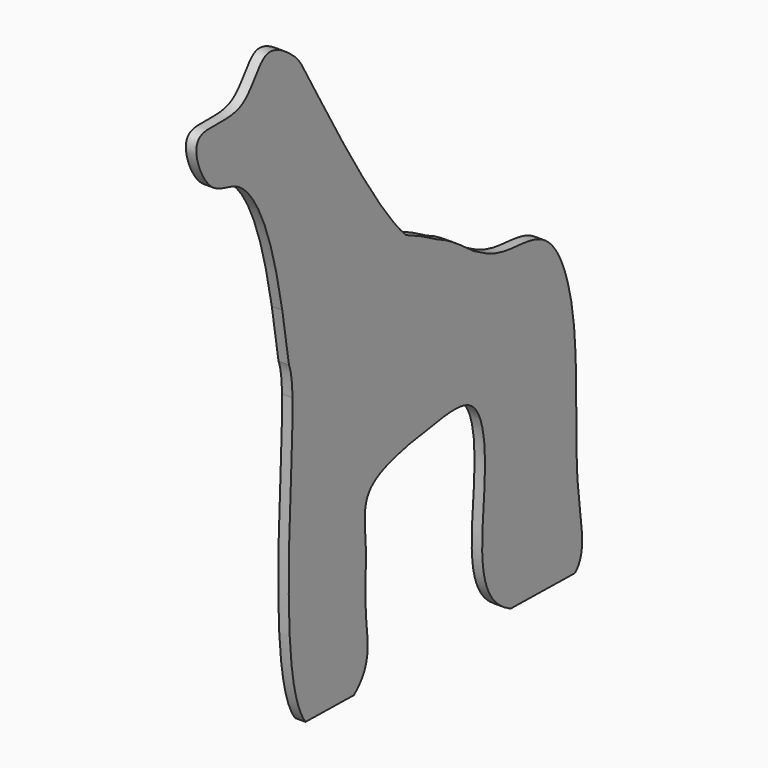
from build123d import *

# Parameters (mm, degrees)
F1_DEPTH = 12


with BuildPart() as f1:
    # F0 (on Right) → F1 (new body)
    with BuildSketch(Plane.YZ):
        with BuildLine():
            add(Edge.make_bspline(
                [(-178.4369833225, -144.2066091912), (-219.218467925, -89.3323742164), (-195.3415795005, 113.7315380775), (-197.007060051, 190.3274804354)],
                knots=[0.0031505946, 0.0031505946, 0.0031505946, 0.0031505946, 0.0998386573, 0.0998386573, 0.0998386573, 0.0998386573], degree=3))
            Line((-178.4369833225, -144.2066091912), (-109.1511381578, -145.4286668255))
            add(Edge.make_bspline(
                [(115.2884357666, -149.3873122617), (107.1403709504, -145.3507189429), (62.2417659614, -114.3804366066), (86.2834183467, -3.0492512147), (70.8695963558, 91.374454728), (0.4418432139, 80.4667572796), (-101.9293868506, 65.0970756202), (-88.6503884924, -2.5844560488), (-96.59431316, -67.481945255), (-83.1150537691, -119.8184104695), (-104.8879154969, -142.055068639), (-109.1511381578, -145.4286668255)],
                knots=[0.6073825493, 0.6073825493, 0.6073825493, 0.6073825493, 0.6195734428, 0.6825204089, 0.7308072739, 0.7727612584, 0.824213165, 0.8635812279, 0.9083971983, 0.9523997564, 0.9613925241, 0.9613925241, 0.9613925241, 0.9613925241], degree=3))
            Line((115.2884357666, -149.3873122617), (207.5685221579, -151.0149402974))
            add(Edge.make_bspline(
                [(63.0940198898, 232.5838804245), (82.5887469223, 220.8525880353), (109.669328549, 211.0698213252), (178.2811116459, 213.9353754027), (217.1880000792, 96.1874140131), (202.5402479992, -58.3272921235), (224.9464188994, -135.8202031967), (207.5685221579, -151.0149402974)],
                knots=[0.3062619929, 0.3062619929, 0.3062619929, 0.3062619929, 0.3456878235, 0.3855453305, 0.441597856, 0.5123533056, 0.5605055591, 0.5605055591, 0.5605055591, 0.5605055591], degree=3))
            add(Edge.make_bspline(
                [(10.2934252514, 265.8684253693), (30.8960203842, 253.7377434197), (48.6497019648, 241.2760009482), (63.0940198898, 232.5838804245)],
                knots=[0.2770500306, 0.2770500306, 0.2770500306, 0.2770500306, 0.3062619929, 0.3062619929, 0.3062619929, 0.3062619929], degree=3))
            add(Edge.make_bspline(
                [(-34.3105899744, 288.3658303985), (-16.0059367898, 270.857218406), (-3.9004302042, 271.3447660229), (10.2934252515, 265.8684253693)],
                knots=[0.8420372945, 0.8420372945, 0.8420372945, 0.8420372945, 0.9166264892, 0.9166264892, 0.9166264892, 0.9166264892], degree=3))
            add(Edge.make_bspline(
                [(-211.7170714071, 284.7467597814), (-184.5213159088, 297.7083735615), (-113.0964050862, 313.28698488), (-53.1463731801, 296.0697503513), (-34.3105899743, 288.3658303985)],
                knots=[0.1907363518, 0.1907363518, 0.1907363518, 0.1907363518, 0.2349239596, 0.2576813871, 0.2576813871, 0.2576813871, 0.2576813871], degree=3))
            add(Edge.make_bspline(
                [(-202.1251185427, 225.6420666888), (-205.1173154703, 245.8230559311), (-208.2397581251, 265.699564879), (-211.7170714094, 284.7467597816)],
                knots=[0.0252319415, 0.0252319415, 0.0252319415, 0.0252319415, 0.0687416948, 0.0687416948, 0.0687416948, 0.0687416948], degree=3))
            add(Edge.make_bspline(
                [(-197.007060051, 190.3274804354), (-197.3715451624, 207.0902583485), (-198.959354649, 217.7959884423), (-202.1251185427, 225.6420666888)],
                knots=[0.0998386573, 0.0998386573, 0.0998386573, 0.0998386573, 0.1209985317, 0.1209985317, 0.1209985317, 0.1209985317], degree=3))
        make_face()
        with BuildLine():
            add(Edge.make_bspline(
                [(-211.7170714094, 284.7467597816), (-217.7643571513, 317.8711350511), (-233.501733701, 385.5372165029), (-270.9766028708, 444.2774273237), (-317.8093852203, 438.6517263777), (-353.310824472, 526.2917032161), (-262.014970167, 495.7742045555), (-241.4702158375, 568.9109908599), (-191.1466514789, 533.2833458738), (-177.7335883136, 511.8222232655), (-76.1302337971, 328.3668022809), (-34.3105899744, 288.3658303985)],
                knots=[0.0687416948, 0.0687416948, 0.0687416948, 0.0687416948, 0.144408133, 0.2359749256, 0.3030161757, 0.3825395321, 0.4642263003, 0.5415325093, 0.6086189201, 0.6716274253, 0.8420372945, 0.8420372945, 0.8420372945, 0.8420372945], degree=3))
            add(Edge.make_bspline(
                [(-211.7170714071, 284.7467597814), (-184.5213159088, 297.7083735615), (-113.0964050862, 313.28698488), (-53.1463731801, 296.0697503513), (-34.3105899743, 288.3658303985)],
                knots=[0.1907363518, 0.1907363518, 0.1907363518, 0.1907363518, 0.2349239596, 0.2576813871, 0.2576813871, 0.2576813871, 0.2576813871], degree=3))
        make_face()
        with BuildLine():
            add(Edge.make_bspline(
                [(10.2934252514, 265.8684253693), (30.8960203842, 253.7377434197), (48.6497019648, 241.2760009482), (63.0940198898, 232.5838804245)],
                knots=[0.2770500306, 0.2770500306, 0.2770500306, 0.2770500306, 0.3062619929, 0.3062619929, 0.3062619929, 0.3062619929], degree=3))
            add(Edge.make_bspline(
                [(10.2934252515, 265.8684253693), (26.1588809193, 259.747139991), (44.6335367378, 246.1745238524), (63.0940198898, 232.5838804245)],
                knots=[0.9166264892, 0.9166264892, 0.9166264892, 0.9166264892, 1, 1, 1, 1], degree=3))
        make_face()
        with BuildLine():
            add(Edge.make_bspline(
                [(-34.3105899743, 288.3658303985), (-18.2796229907, 281.8090928814), (-3.3668798977, 273.9115294555), (10.2934252514, 265.8684253693)],
                knots=[0.2576813871, 0.2576813871, 0.2576813871, 0.2576813871, 0.2770500306, 0.2770500306, 0.2770500306, 0.2770500306], degree=3))
            add(Edge.make_bspline(
                [(-34.3105899744, 288.3658303985), (-16.0059367898, 270.857218406), (-3.9004302042, 271.3447660229), (10.2934252515, 265.8684253693)],
                knots=[0.8420372945, 0.8420372945, 0.8420372945, 0.8420372945, 0.9166264892, 0.9166264892, 0.9166264892, 0.9166264892], degree=3))
        make_face()
    extrude(amount=F1_DEPTH)


solid = f1.part
